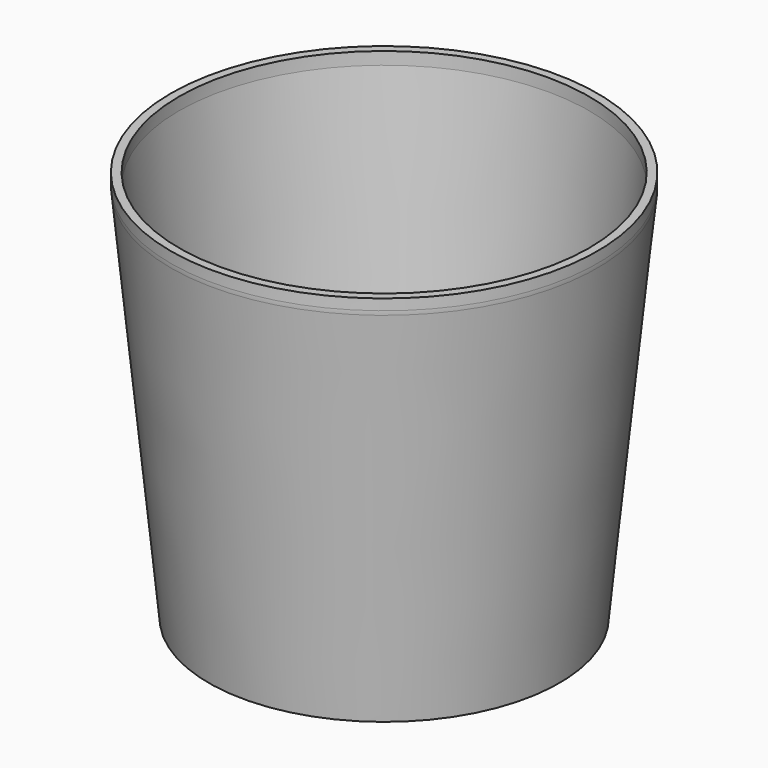
from build123d import *

# Parameters (mm, degrees)
F3_DEPTH = 2.001


with BuildPart() as f1:
    # F0 (on Front) → F1 (revolve)
    with BuildSketch(Plane.XZ):
        with BuildLine():
            Line((-41.9872180451, 0), (-31.5, 0))
            Line((-31.5, 0), (-31.5, 2))
            Line((-31.5, 2), (-35.6538847118, 2))
            ThreePointArc((-35.6538847118, 2), (-39.0084513316, 3.2923211044), (-40.6289470559, 6.5012468828))
            Line((-40.6289470559, 6.5012468828), (-49.1, 91))
            Line((-49.1, 91), (-49.1, 94))
            Line((-49.1, 94), (-51.1, 94))
            Line((-51.1, 94), (-51.1, 91.4))
            ThreePointArc((-51.1, 91.4), (-51.0875233888, 90.9006238306), (-51.0501246883, 90.4024937656))
            Line((-51.0501246883, 90.4024937656), (-41.9872180451, 0))
        make_face()
    revolve(axis=Axis((0, 0, -11.3997804001), (0, 0, -1)))

    # F2 (on face) → F3 (cut, through all)
    with BuildSketch(Plane.XY.offset(2)):
        with BuildLine():
            ThreePointArc((31.5, 0), (31.4841069455, -1.0005047961), (31.4364438192, -2))
            ThreePointArc((31.4364438192, -2), (33.4364438192, 0), (31.4364438192, 2))
            ThreePointArc((31.4364438192, 2), (31.4841069455, 1.0005047961), (31.5, 0))
        make_face()
    extrude(amount=-F3_DEPTH, mode=Mode.SUBTRACT)


solid = f1.part
